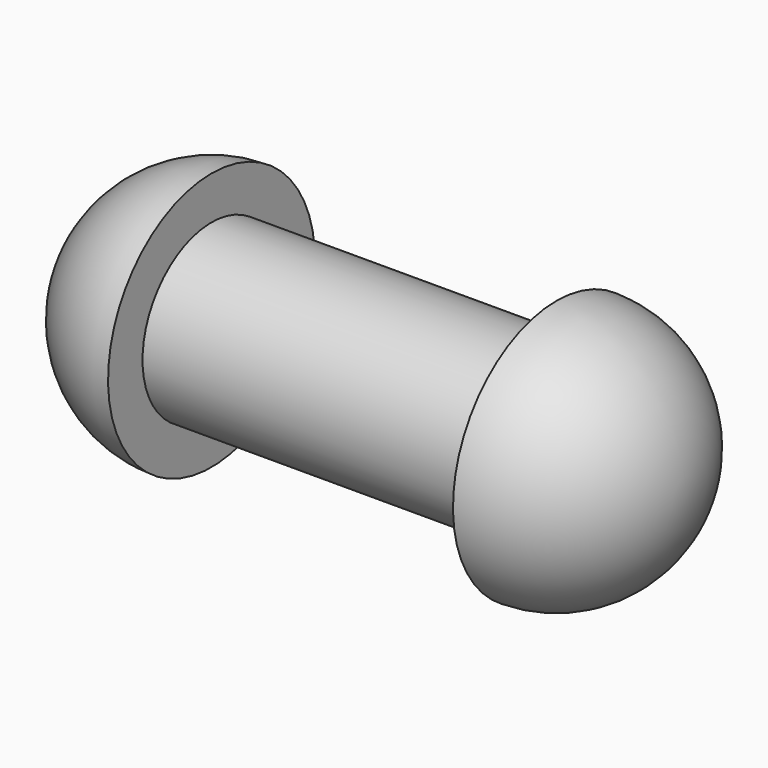
from build123d import *

# Parameters (mm, degrees)
F0_R     = 1
F1_DEPTH = 2


# Not quite as in the source:
# - a pattern or mirror of a feature is missing from the dataset's text; its kind, count and spacing are read off the source's solid


with BuildPart() as f1:
    # F0 (on Right) → F1 (new body, symmetric)
    with BuildSketch(Plane.YZ):
        Circle(F0_R)
    extrude(amount=F1_DEPTH, both=True)

    # F2 (on Front) → F3 (revolve)
    with BuildSketch(Plane.XZ):
        with BuildLine():
            Line((2, 0), (3.5, 0))
            ThreePointArc((3.5, 0), (3.0606601718, 1.0606601718), (2, 1.5))
            Line((2, 1.5), (2, 0))
        make_face()
    f3 = revolve(axis=Axis((2, 0, 0), (1, 0, 0)))

    # F3_copies: F3 across plane
    add(f3.mirror(Plane(origin=(0, 0, 0), x_dir=(0, 0, -1), z_dir=(-1, 0, 0))))


solid = f1.part
